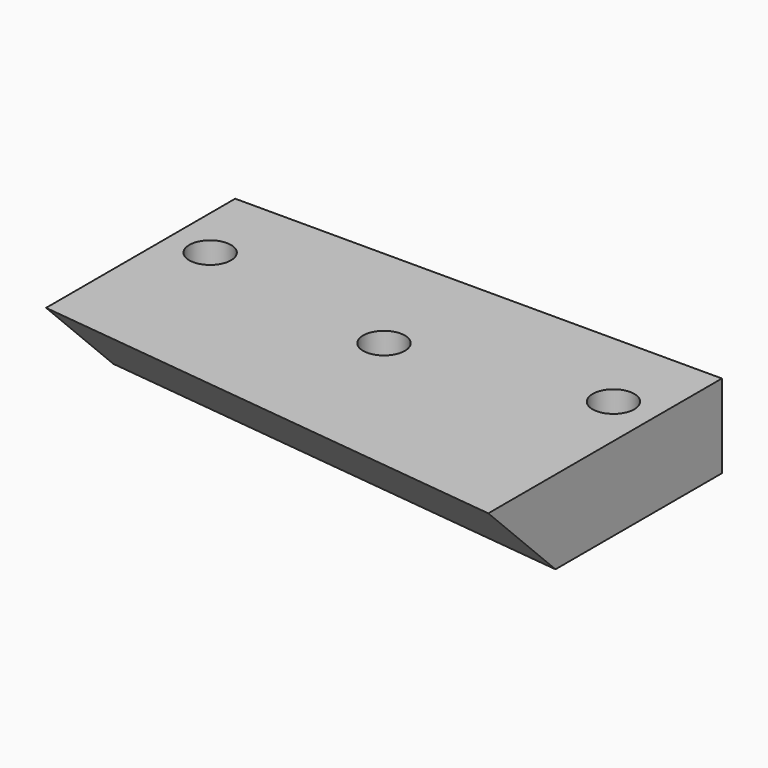
from build123d import *

# Parameters (mm, degrees)
F1_DEPTH = 6
F2_SIZE  = 5.99999
F3_R     = 1.5
F4_DEPTH = 6


# Not quite as in the source:
# - a fillet or chamfer is up to 0.001 mm smaller than in the source, because OpenCascade refuses the exact size


with BuildPart() as f1:
    # F0 (on Top) → F1 (new body)
    with BuildSketch(Plane.XY):
        Polygon((31.2662842423, 6.9127185345), (-3.7337157577, 6.9127185345), (-3.7337157577, -10.0872814655), (31.2662842423, -14.0872814655), align=None)
    extrude(amount=F1_DEPTH)

    # F2 (size 6 in the source; OpenCascade refuses exactly that, so slightly less here)
    f2_edges = [f1.edges().sort_by_distance(p)[0] for p in [
        (13.766284, -12.087281, 0),
    ]]
    chamfer(f2_edges, length=F2_SIZE)

    # F3 (on face) → F4 (cut, through all)
    with BuildSketch(Plane.XY.offset(6)):
        with Locations((-0.7337157577, 0.9127185345)):
            Circle(F3_R)
        with Locations((13.7662842423, -1.5872814655)):
            Circle(F3_R)
        with Locations((28.2662842423, 0.9127185345)):
            Circle(F3_R)
    extrude(amount=-F4_DEPTH, mode=Mode.SUBTRACT)


solid = f1.part
